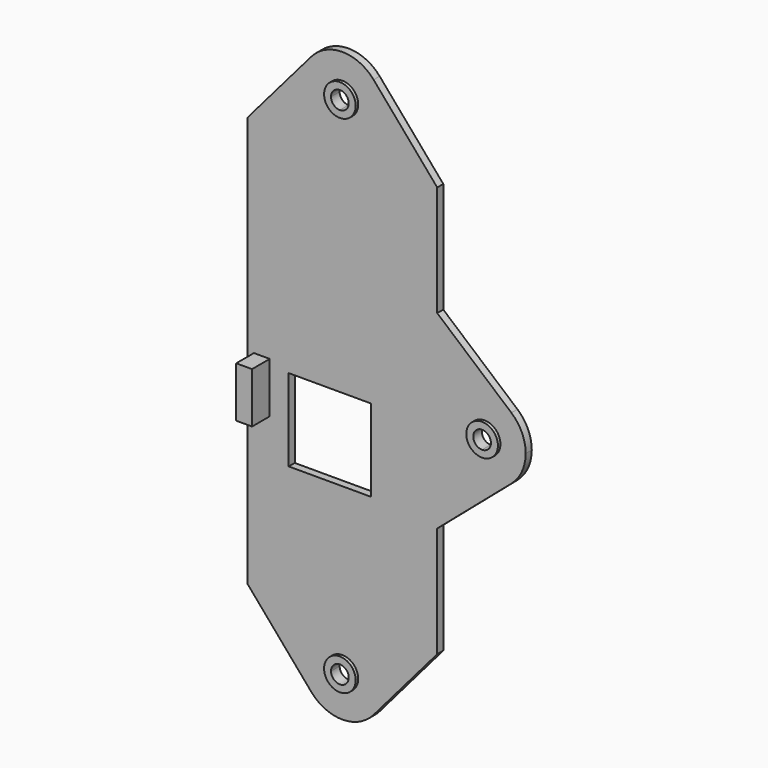
from build123d import *

# Parameters (mm, degrees)
F1_DEPTH = 1.2
F2_DEPTH = 1.7
F0_W     = 2.5
F0_H     = 8
F3_DEPTH = 4.7


with BuildPart() as f1:
    # F0 (on Front) → F1 (new body)
    with BuildSketch(Plane.XZ):
        Polygon((-6.3577895987, -1.8137509867), (-6.3577895987, 30.6862490133), (-12.8577895987, 30.6862490133), (-21.3577895987, 30.6862490133), (-21.3577895987, -1.8137509867), (-20.3577895987, -1.8137509867), (-17.8577895987, -1.8137509867), align=None)
        Polygon((0.1422104013, 30.6862490133), (-6.3577895987, 30.6862490133), (-6.3577895987, -1.8137509867), (8.6422104013, -1.8137509867), (8.6422104013, -0.8137509867), (8.6422104013, 4.6862490133), (8.6422104013, 13.1862490133), (8.6422104013, 30.6862490133), align=None)
        with BuildLine():
            Line((-21.3577895987, 30.6862490133), (-12.8577895987, 30.6862490133))
            Line((-12.8577895987, 30.6862490133), (-12.8577895987, 38.1862490133))
            ThreePointArc((-12.8577895987, 38.1862490133), (-12.4534647314, 40.4429600442), (-11.2907912366, 42.4189189557))
            Line((-11.2907912366, 42.4189189557), (-21.3577895987, 30.6862490133))
        make_face()
        with BuildLine():
            Line((0.1422104013, 38.1862490133), (0.1422104013, 30.6862490133))
            Line((0.1422104013, 30.6862490133), (8.6422104013, 30.6862490133))
            Line((8.6422104013, 30.6862490133), (-1.4247879609, 42.4189189557))
            ThreePointArc((-1.4247879609, 42.4189189557), (-0.2621144661, 40.4429600442), (0.1422104013, 38.1862490133))
        make_face()
        Polygon((8.6422104013, -1.8137509867), (-6.3577895987, -1.8137509867), (-6.3577895987, -2.8137509867), (-1.8577895987, -2.8137509867), (-1.8577895987, -15.8137509867), (-6.3577895987, -15.8137509867), (-6.3577895987, -34.3137509867), (0.1422104013, -34.3137509867), (8.6422104013, -34.3137509867), (8.6422104013, -16.8137509867), (8.6422104013, -8.3137509867), align=None)
        Polygon((-6.3577895987, -2.8137509867), (-6.3577895987, -1.8137509867), (-17.8577895987, -1.8137509867), (-17.8577895987, -9.8137509867), (-20.3577895987, -9.8137509867), (-20.3577895987, -1.8137509867), (-21.3577895987, -1.8137509867), (-21.3577895987, -34.3137509867), (-12.8577895987, -34.3137509867), (-6.3577895987, -34.3137509867), (-6.3577895987, -15.8137509867), (-14.8577895987, -15.8137509867), (-14.8577895987, -2.8137509867), align=None)
        with BuildLine():
            ThreePointArc((-11.2907912366, 42.4189189557), (-12.4534647314, 40.4429600442), (-12.8577895987, 38.1862490133))
            Line((-12.8577895987, 38.1862490133), (-8.8577895987, 38.1862490133))
            ThreePointArc((-8.8577895987, 38.1862490133), (-6.3577895987, 40.6862490133), (-3.8577895987, 38.1862490133))
            Line((-3.8577895987, 38.1862490133), (0.1422104013, 38.1862490133))
            ThreePointArc((0.1422104013, 38.1862490133), (-0.2621144661, 40.4429600442), (-1.4247879609, 42.4189189557))
            ThreePointArc((-1.4247879609, 42.4189189557), (-6.3577895987, 44.6862490133), (-11.2907912366, 42.4189189557))
        make_face()
        with BuildLine():
            Line((20.3748803436, 3.1192506512), (8.6422104013, 13.1862490133))
            Line((8.6422104013, 13.1862490133), (8.6422104013, 4.6862490133))
            Line((8.6422104013, 4.6862490133), (16.1422104013, 4.6862490133))
            ThreePointArc((16.1422104013, 4.6862490133), (18.3989214322, 4.281924146), (20.3748803436, 3.1192506512))
        make_face()
        with BuildLine():
            Line((16.1422104013, -8.3137509867), (8.6422104013, -8.3137509867))
            Line((8.6422104013, -8.3137509867), (8.6422104013, -16.8137509867))
            Line((8.6422104013, -16.8137509867), (20.3748803436, -6.7467526245))
            ThreePointArc((20.3748803436, -6.7467526245), (18.3989214322, -7.9094261194), (16.1422104013, -8.3137509867))
        make_face()
        with BuildLine():
            Line((-12.8577895987, -34.3137509867), (-21.3577895987, -34.3137509867))
            Line((-21.3577895987, -34.3137509867), (-11.290791296, -46.0464208599))
            ThreePointArc((-11.290791296, -46.0464208599), (-12.4534647472, -44.0704619748), (-12.8577895987, -41.8137509867))
            Line((-12.8577895987, -41.8137509867), (-12.8577895987, -34.3137509867))
        make_face()
        with BuildLine():
            ThreePointArc((22.6422104013, -1.8137509867), (22.0482392966, 0.9008065624), (20.3748803436, 3.1192506512))
            ThreePointArc((20.3748803436, 3.1192506512), (18.3989214322, 4.281924146), (16.1422104013, 4.6862490133))
            Line((16.1422104013, 4.6862490133), (16.1422104013, 0.6862490133))
            ThreePointArc((16.1422104013, 0.6862490133), (17.9099773542, -0.0459840337), (18.6422104013, -1.8137509867))
            ThreePointArc((18.6422104013, -1.8137509867), (17.9099773542, -3.5815179397), (16.1422104013, -4.3137509867))
            Line((16.1422104013, -4.3137509867), (16.1422104013, -8.3137509867))
            ThreePointArc((16.1422104013, -8.3137509867), (18.3989214322, -7.9094261194), (20.3748803436, -6.7467526245))
            ThreePointArc((20.3748803436, -6.7467526245), (22.0482392966, -4.5283085358), (22.6422104013, -1.8137509867))
        make_face()
        with BuildLine():
            ThreePointArc((-12.8577895987, -41.8137509867), (-12.4534647472, -44.0704619748), (-11.290791296, -46.0464208599))
            ThreePointArc((-11.290791296, -46.0464208599), (-6.3577896443, -48.3137509867), (-1.4247879609, -46.0464209291))
            ThreePointArc((-1.4247879609, -46.0464209291), (-0.2621144661, -44.0704620176), (0.1422104013, -41.8137509867))
            Line((0.1422104013, -41.8137509867), (-3.8577895987, -41.8137509867))
            ThreePointArc((-3.8577895987, -41.8137509867), (-6.3577895987, -44.3137509867), (-8.8577895987, -41.8137509867))
            Line((-8.8577895987, -41.8137509867), (-12.8577895987, -41.8137509867))
        make_face()
        with BuildLine():
            Line((8.6422104013, -34.3137509867), (0.1422104013, -34.3137509867))
            Line((0.1422104013, -34.3137509867), (0.1422104013, -41.8137509867))
            ThreePointArc((0.1422104013, -41.8137509867), (-0.2621144661, -44.0704620176), (-1.4247879609, -46.0464209291))
            Line((-1.4247879609, -46.0464209291), (8.6422104013, -34.3137509867))
        make_face()
        with BuildLine():
            ThreePointArc((-12.8577895987, 38.1862490133), (-10.9539836765, 33.5900549356), (-6.3577895987, 31.6862490133))
            Line((-6.3577895987, 31.6862490133), (-6.3577895987, 35.6862490133))
            ThreePointArc((-6.3577895987, 35.6862490133), (-8.1255565517, 36.4184820603), (-8.8577895987, 38.1862490133))
            Line((-8.8577895987, 38.1862490133), (-12.8577895987, 38.1862490133))
        make_face()
        with BuildLine():
            Line((-12.8577895987, 30.6862490133), (-6.3577895987, 30.6862490133))
            Line((-6.3577895987, 30.6862490133), (-6.3577895987, 31.6862490133))
            ThreePointArc((-6.3577895987, 31.6862490133), (-10.9539836765, 33.5900549356), (-12.8577895987, 38.1862490133))
            Line((-12.8577895987, 38.1862490133), (-12.8577895987, 30.6862490133))
        make_face()
        with BuildLine():
            Line((13.6422104013, -1.8137509867), (9.6422104013, -1.8137509867))
            ThreePointArc((9.6422104013, -1.8137509867), (11.5460163235, -6.4099450644), (16.1422104013, -8.3137509867))
            Line((16.1422104013, -8.3137509867), (16.1422104013, -4.3137509867))
            ThreePointArc((16.1422104013, -4.3137509867), (14.3744434483, -3.5815179397), (13.6422104013, -1.8137509867))
        make_face()
        with BuildLine():
            Line((8.6422104013, 4.6862490133), (8.6422104013, -0.8137509867))
            Line((8.6422104013, -0.8137509867), (9.7195941119, -0.8137509867))
            ThreePointArc((9.7195941119, -0.8137509867), (11.9143267699, 3.1233534278), (16.1422104013, 4.6862490133))
            Line((16.1422104013, 4.6862490133), (8.6422104013, 4.6862490133))
        make_face()
        with BuildLine():
            Line((0.1422104013, -34.3137509867), (-6.3577895987, -34.3137509867))
            Line((-6.3577895987, -34.3137509867), (-6.3577895987, -35.3137509867))
            ThreePointArc((-6.3577895987, -35.3137509867), (-1.761595521, -37.217556909), (0.1422104013, -41.8137509867))
            Line((0.1422104013, -41.8137509867), (0.1422104013, -34.3137509867))
        make_face()
        with BuildLine():
            Line((-6.3577895987, -35.3137509867), (-6.3577895987, -34.3137509867))
            Line((-6.3577895987, -34.3137509867), (-12.8577895987, -34.3137509867))
            Line((-12.8577895987, -34.3137509867), (-12.8577895987, -41.8137509867))
            ThreePointArc((-12.8577895987, -41.8137509867), (-10.9539836765, -37.217556909), (-6.3577895987, -35.3137509867))
        make_face()
        with BuildLine():
            Line((-6.3577895987, -39.3137509867), (-6.3577895987, -35.3137509867))
            ThreePointArc((-6.3577895987, -35.3137509867), (-10.9539836765, -37.217556909), (-12.8577895987, -41.8137509867))
            Line((-12.8577895987, -41.8137509867), (-8.8577895987, -41.8137509867))
            ThreePointArc((-8.8577895987, -41.8137509867), (-8.1255565517, -40.0459840337), (-6.3577895987, -39.3137509867))
        make_face()
        with BuildLine():
            ThreePointArc((0.1422104013, -41.8137509867), (-1.761595521, -37.217556909), (-6.3577895987, -35.3137509867))
            Line((-6.3577895987, -35.3137509867), (-6.3577895987, -39.3137509867))
            ThreePointArc((-6.3577895987, -39.3137509867), (-4.5900226458, -40.0459840337), (-3.8577895987, -41.8137509867))
            Line((-3.8577895987, -41.8137509867), (0.1422104013, -41.8137509867))
        make_face()
        with BuildLine():
            Line((-6.3577895987, 31.6862490133), (-6.3577895987, 30.6862490133))
            Line((-6.3577895987, 30.6862490133), (0.1422104013, 30.6862490133))
            Line((0.1422104013, 30.6862490133), (0.1422104013, 38.1862490133))
            ThreePointArc((0.1422104013, 38.1862490133), (-1.761595521, 33.5900549356), (-6.3577895987, 31.6862490133))
        make_face()
        with BuildLine():
            Line((-6.3577895987, 35.6862490133), (-6.3577895987, 31.6862490133))
            ThreePointArc((-6.3577895987, 31.6862490133), (-1.761595521, 33.5900549356), (0.1422104013, 38.1862490133))
            Line((0.1422104013, 38.1862490133), (-3.8577895987, 38.1862490133))
            ThreePointArc((-3.8577895987, 38.1862490133), (-4.5900226458, 36.4184820603), (-6.3577895987, 35.6862490133))
        make_face()
        with BuildLine():
            Line((9.6422104013, -1.8137509867), (8.6422104013, -1.8137509867))
            Line((8.6422104013, -1.8137509867), (8.6422104013, -8.3137509867))
            Line((8.6422104013, -8.3137509867), (16.1422104013, -8.3137509867))
            ThreePointArc((16.1422104013, -8.3137509867), (11.5460163235, -6.4099450644), (9.6422104013, -1.8137509867))
        make_face()
        with BuildLine():
            ThreePointArc((16.1422104013, 4.6862490133), (11.9143267699, 3.1233534278), (9.7195941119, -0.8137509867))
            Line((9.7195941119, -0.8137509867), (13.8509225538, -0.8137509867))
            ThreePointArc((13.8509225538, -0.8137509867), (14.7729040075, 0.2778990796), (16.1422104013, 0.6862490133))
            Line((16.1422104013, 0.6862490133), (16.1422104013, 4.6862490133))
        make_face()
        with BuildLine():
            ThreePointArc((9.7195941119, -0.8137509867), (9.6615852045, -1.3122561615), (9.6422104013, -1.8137509867))
            Line((9.6422104013, -1.8137509867), (13.6422104013, -1.8137509867))
            ThreePointArc((13.6422104013, -1.8137509867), (13.6949446189, -1.3029768775), (13.8509225538, -0.8137509867))
            Line((13.8509225538, -0.8137509867), (9.7195941119, -0.8137509867))
        make_face()
        with BuildLine():
            Line((8.6422104013, -0.8137509867), (8.6422104013, -1.8137509867))
            Line((8.6422104013, -1.8137509867), (9.6422104013, -1.8137509867))
            ThreePointArc((9.6422104013, -1.8137509867), (9.6615852045, -1.3122561615), (9.7195941119, -0.8137509867))
            Line((9.7195941119, -0.8137509867), (8.6422104013, -0.8137509867))
        make_face()
    extrude(amount=F1_DEPTH)

    # F0 (on Front) → F2 (join)
    with BuildSketch(Plane.XZ):
        with BuildLine():
            Line((-6.3577895987, 36.7862490133), (-6.3577895987, 35.6862490133))
            ThreePointArc((-6.3577895987, 35.6862490133), (-4.5900226458, 36.4184820603), (-3.8577895987, 38.1862490133))
            Line((-3.8577895987, 38.1862490133), (-4.9577895987, 38.1862490133))
            ThreePointArc((-4.9577895987, 38.1862490133), (-5.3678401051, 37.1962995197), (-6.3577895987, 36.7862490133))
        make_face()
        with BuildLine():
            ThreePointArc((-3.8577895987, 38.1862490133), (-6.3577895987, 40.6862490133), (-8.8577895987, 38.1862490133))
            Line((-8.8577895987, 38.1862490133), (-7.7577895987, 38.1862490133))
            ThreePointArc((-7.7577895987, 38.1862490133), (-6.3577895987, 39.5862490133), (-4.9577895987, 38.1862490133))
            Line((-4.9577895987, 38.1862490133), (-3.8577895987, 38.1862490133))
        make_face()
        with BuildLine():
            ThreePointArc((-8.8577895987, 38.1862490133), (-8.1255565517, 36.4184820603), (-6.3577895987, 35.6862490133))
            Line((-6.3577895987, 35.6862490133), (-6.3577895987, 36.7862490133))
            ThreePointArc((-6.3577895987, 36.7862490133), (-7.3477390924, 37.1962995197), (-7.7577895987, 38.1862490133))
            Line((-7.7577895987, 38.1862490133), (-8.8577895987, 38.1862490133))
        make_face()
        with BuildLine():
            Line((14.7422104013, -1.8137509867), (13.6422104013, -1.8137509867))
            ThreePointArc((13.6422104013, -1.8137509867), (14.3744434483, -3.5815179397), (16.1422104013, -4.3137509867))
            Line((16.1422104013, -4.3137509867), (16.1422104013, -3.2137509867))
            ThreePointArc((16.1422104013, -3.2137509867), (15.1522609076, -2.8037004803), (14.7422104013, -1.8137509867))
        make_face()
        with BuildLine():
            Line((16.1422104013, -3.2137509867), (16.1422104013, -4.3137509867))
            ThreePointArc((16.1422104013, -4.3137509867), (17.9099773542, -3.5815179397), (18.6422104013, -1.8137509867))
            ThreePointArc((18.6422104013, -1.8137509867), (17.9099773542, -0.0459840337), (16.1422104013, 0.6862490133))
            Line((16.1422104013, 0.6862490133), (16.1422104013, -0.4137509867))
            ThreePointArc((16.1422104013, -0.4137509867), (17.1321598949, -0.823801493), (17.5422104013, -1.8137509867))
            ThreePointArc((17.5422104013, -1.8137509867), (17.1321598949, -2.8037004803), (16.1422104013, -3.2137509867))
        make_face()
        with BuildLine():
            Line((-7.7577895987, -41.8137509867), (-8.8577895987, -41.8137509867))
            ThreePointArc((-8.8577895987, -41.8137509867), (-6.3577895987, -44.3137509867), (-3.8577895987, -41.8137509867))
            Line((-3.8577895987, -41.8137509867), (-4.9577895987, -41.8137509867))
            ThreePointArc((-4.9577895987, -41.8137509867), (-6.3577895987, -43.2137509867), (-7.7577895987, -41.8137509867))
        make_face()
        with BuildLine():
            Line((-6.3577895987, -40.4137509867), (-6.3577895987, -39.3137509867))
            ThreePointArc((-6.3577895987, -39.3137509867), (-8.1255565517, -40.0459840337), (-8.8577895987, -41.8137509867))
            Line((-8.8577895987, -41.8137509867), (-7.7577895987, -41.8137509867))
            ThreePointArc((-7.7577895987, -41.8137509867), (-7.3477390924, -40.823801493), (-6.3577895987, -40.4137509867))
        make_face()
        with BuildLine():
            ThreePointArc((-3.8577895987, -41.8137509867), (-4.5900226458, -40.0459840337), (-6.3577895987, -39.3137509867))
            Line((-6.3577895987, -39.3137509867), (-6.3577895987, -40.4137509867))
            ThreePointArc((-6.3577895987, -40.4137509867), (-5.3678401051, -40.823801493), (-4.9577895987, -41.8137509867))
            Line((-4.9577895987, -41.8137509867), (-3.8577895987, -41.8137509867))
        make_face()
        with BuildLine():
            ThreePointArc((16.1422104013, 0.6862490133), (14.7729040075, 0.2778990796), (13.8509225538, -0.8137509867))
            Line((13.8509225538, -0.8137509867), (15.1624145041, -0.8137509867))
            ThreePointArc((15.1624145041, -0.8137509867), (15.613060139, -0.517602847), (16.1422104013, -0.4137509867))
            Line((16.1422104013, -0.4137509867), (16.1422104013, 0.6862490133))
        make_face()
        with BuildLine():
            ThreePointArc((13.8509225538, -0.8137509867), (13.6949446189, -1.3029768775), (13.6422104013, -1.8137509867))
            Line((13.6422104013, -1.8137509867), (14.7422104013, -1.8137509867))
            ThreePointArc((14.7422104013, -1.8137509867), (14.8515295236, -1.2714015864), (15.1624145041, -0.8137509867))
            Line((15.1624145041, -0.8137509867), (13.8509225538, -0.8137509867))
        make_face()
    extrude(amount=F2_DEPTH)

    # F0 (on Front) → F3 (join)
    with BuildSketch(Plane.XZ):
        with Locations((-19.1077895987, -5.8137509867)):
            Rectangle(F0_W, F0_H)
    extrude(amount=F3_DEPTH)


solid = f1.part
